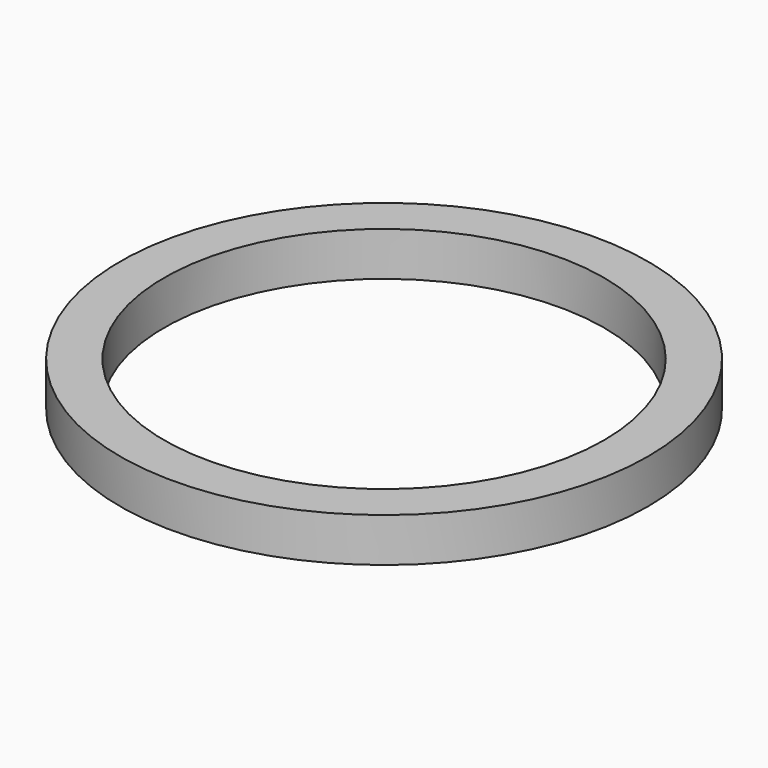
from build123d import *

# Parameters (mm, degrees)
F0_R     = 18
F0_R_2   = 15
F1_DEPTH = 3


# Not quite as in the source:
# - the program builds the solid bodies; features that only make, move or delete a surface that nothing else refers to are left out


with BuildPart() as f1:
    # F0 (on Top) → F1 (new body)
    with BuildSketch(Plane.XY):
        Circle(F0_R)
        Circle(F0_R_2, mode=Mode.SUBTRACT)
    extrude(amount=F1_DEPTH)


solid = f1.part
